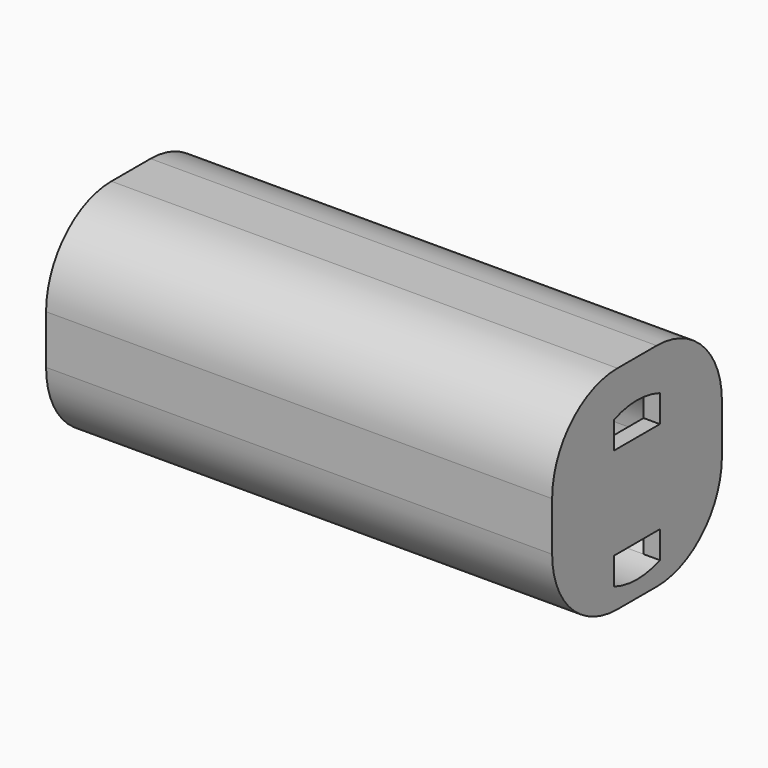
from build123d import *

# Parameters (mm, degrees)
F0_W        = 39
F0_H        = 39
F0_R        = 16.5
F1_DEPTH    = 90
F0_R_2      = 2
F2_DEPTH    = 3
F3_W        = 75
F3_H        = 23
F4_DEPTH    = 21.5
F5_DEPTH    = 10
F6_T1_DEPTH = 127.5
F6_T3_DEPTH = 40.5


# Not quite as in the source:
# - a fillet or chamfer that OpenCascade refuses, or shapes differently, is made with other operations: its cross-section is extruded or revolved along the edge and cut away or added
# - a feature names something its author has since deleted; it is built from what else it names


with BuildPart() as f1:
    # F0 (on Right) → F1 (new body)
    with BuildSketch(Plane.YZ):
        with Locations((0, 2)):
            Rectangle(F0_W, F0_H)
        Circle(F0_R, mode=Mode.SUBTRACT)
        Circle(F0_R)
        with BuildLine():
            ThreePointArc((5.25, 13.5161939909), (11.9660979438, 8.1891696771), (14.5, 0))
            ThreePointArc((14.5, 0), (11.9660979438, -8.1891696771), (5.25, -13.5161939909))
            ThreePointArc((5.25, -13.5161939909), (0, -14.5), (-5.25, -13.5161939909))
            ThreePointArc((-5.25, -13.5161939909), (-14.5, 0), (-5.25, 13.5161939909))
            ThreePointArc((-5.25, 13.5161939909), (0, 14.5), (5.25, 13.5161939909))
        make_face(mode=Mode.SUBTRACT)
    extrude(amount=-F1_DEPTH)

    # F0 (on Right) → F2 (join)
    with BuildSketch(Plane.YZ):
        with Locations((0, 2)):
            Rectangle(F0_W, F0_H)
        Circle(F0_R, mode=Mode.SUBTRACT)
        Circle(F0_R)
        with BuildLine():
            ThreePointArc((5.25, 13.5161939909), (11.9660979438, 8.1891696771), (14.5, 0))
            ThreePointArc((14.5, 0), (11.9660979438, -8.1891696771), (5.25, -13.5161939909))
            ThreePointArc((5.25, -13.5161939909), (0, -14.5), (-5.25, -13.5161939909))
            ThreePointArc((-5.25, -13.5161939909), (-14.5, 0), (-5.25, 13.5161939909))
            ThreePointArc((-5.25, 13.5161939909), (0, 14.5), (5.25, 13.5161939909))
        make_face(mode=Mode.SUBTRACT)
        with BuildLine():
            ThreePointArc((5.25, -13.5161939909), (11.9660979438, -8.1891696771), (14.5, 0))
            ThreePointArc((14.5, 0), (11.9660979438, 8.1891696771), (5.25, 13.5161939909))
            Line((5.25, 13.5161939909), (5.25, 8.5))
            Line((5.25, 8.5), (-5.25, 8.5))
            Line((-5.25, 8.5), (-5.25, 13.5161939909))
            ThreePointArc((-5.25, 13.5161939909), (-14.5, 0), (-5.25, -13.5161939909))
            Line((-5.25, -13.5161939909), (-5.25, -8.5))
            Line((-5.25, -8.5), (5.25, -8.5))
            Line((5.25, -8.5), (5.25, -13.5161939909))
        make_face()
        Circle(F0_R_2, mode=Mode.SUBTRACT)
        Circle(F0_R_2)
    extrude(amount=F2_DEPTH)

    # F3 (on face) → F4 (cut)
    with BuildSketch(Plane(origin=(0, 0, -17.5), x_dir=(1, 0, 0), z_dir=(0, 0, -1))):
        with Locations((-44.5, 0)):
            Rectangle(F3_W, F3_H)
    extrude(amount=-F4_DEPTH, mode=Mode.SUBTRACT)

    # F0 (on Right) → F5 (join)
    with BuildSketch(Plane.YZ):
        Circle(F0_R_2)
    extrude(amount=-F5_DEPTH)

    # F6: fillet of radius 15 on 8 edges, made by hand

    # F6_s2 → F6_t1 (cut)
    with BuildSketch(Plane.YZ.offset(-127.5)):
        with BuildLine():
            ThreePointArc((4.5, -17.5), (15.1066017178, -13.1066017178), (19.5, -2.5))
            Line((19.5, -2.5), (19.5, -17.5))
            Line((19.5, -17.5), (4.5, -17.5))
        make_face()
        with BuildLine():
            ThreePointArc((-19.5, -2.5), (-15.1066017178, -13.1066017178), (-4.5, -17.5))
            Line((-4.5, -17.5), (-19.5, -17.5))
            Line((-19.5, -17.5), (-19.5, -2.5))
        make_face()
        with BuildLine():
            ThreePointArc((4.5, 21.5), (15.1066017178, 17.1066017178), (19.5, 6.5))
            Line((19.5, 6.5), (19.5, 21.5))
            Line((19.5, 21.5), (4.5, 21.5))
        make_face()
        with BuildLine():
            ThreePointArc((-4.5, 21.5), (-15.1066017178, 17.1066017178), (-19.5, 6.5))
            Line((-19.5, 6.5), (-19.5, 21.5))
            Line((-19.5, 21.5), (-4.5, 21.5))
        make_face()
    extrude(amount=F6_T1_DEPTH, mode=Mode.SUBTRACT)

    # F6_s4 → F6_t3 (cut)
    with BuildSketch(Plane.YZ):
        with BuildLine():
            ThreePointArc((4.5, -17.5), (15.1066017178, -13.1066017178), (19.5, -2.5))
            Line((19.5, -2.5), (19.5, -17.5))
            Line((19.5, -17.5), (4.5, -17.5))
        make_face()
        with BuildLine():
            ThreePointArc((-19.5, -2.5), (-15.1066017178, -13.1066017178), (-4.5, -17.5))
            Line((-4.5, -17.5), (-19.5, -17.5))
            Line((-19.5, -17.5), (-19.5, -2.5))
        make_face()
        with BuildLine():
            ThreePointArc((4.5, 21.5), (15.1066017178, 17.1066017178), (19.5, 6.5))
            Line((19.5, 6.5), (19.5, 21.5))
            Line((19.5, 21.5), (4.5, 21.5))
        make_face()
        with BuildLine():
            ThreePointArc((-4.5, 21.5), (-15.1066017178, 17.1066017178), (-19.5, 6.5))
            Line((-19.5, 6.5), (-19.5, 21.5))
            Line((-19.5, 21.5), (-4.5, 21.5))
        make_face()
    extrude(amount=F6_T3_DEPTH, mode=Mode.SUBTRACT)


solid = f1.part
